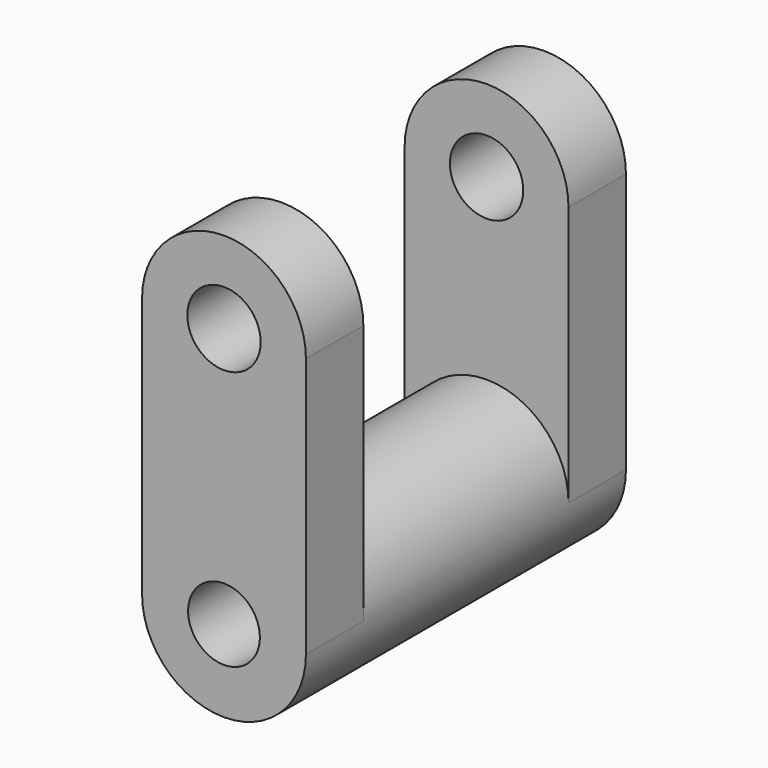
from build123d import *

# Parameters (mm, degrees)
F0_R     = 11.3530222264
F1_DEPTH = 22.225
F4_DEPTH = 79.375
F6_D     = 22.225


with BuildPart() as f1:
    # F0 (on Front) → F1 (new body)
    with BuildSketch(Plane.XZ):
        with BuildLine():
            Line((25.3637172282, -40.2771420777), (25.3637172282, 40.2771420777))
            ThreePointArc((25.3637172282, 40.2771420777), (0, 65.6408593059), (-25.3637172282, 40.2771420777))
            Line((-25.3637172282, 40.2771420777), (-25.3637172282, -40.2771420777))
            ThreePointArc((-25.3637172282, -40.2771420777), (0, -65.6408593059), (25.3637172282, -40.2771420777))
        make_face()
        with Locations((0, 40.2771420777)):
            Circle(F0_R, mode=Mode.SUBTRACT)
    extrude(amount=F1_DEPTH)


with BuildPart() as f2_1:
    # F2: copy of F1
    add(f1.part.moved(Location((0, 101.6, 0))))


with BuildPart() as f1_1:
    add(f1.part)

    add(f2_1.part)  # F4 merges F2_1
    # F3 (on face) → F4 (join, through all)
    with BuildSketch(Plane(origin=(0, 0, 0), x_dir=(-1, 0, 0), z_dir=(0, 1, 0))):
        with BuildLine():
            ThreePointArc((-25.3637172282, -40.2771420777), (0, -65.6408593059), (25.3637172282, -40.2771420777))
            ThreePointArc((25.3637172282, -40.2771420777), (0, -14.9134248495), (-25.3637172282, -40.2771420777))
        make_face()
    extrude(amount=F4_DEPTH)

    # F6 (through all)
    with Locations(Plane(origin=(0, 101.6, 0), x_dir=(-1, 0, 0), z_dir=(0, 1, 0))):
        with Locations((0, -40.2771420777)):
            Hole(F6_D / 2)


solid = f1_1.part
